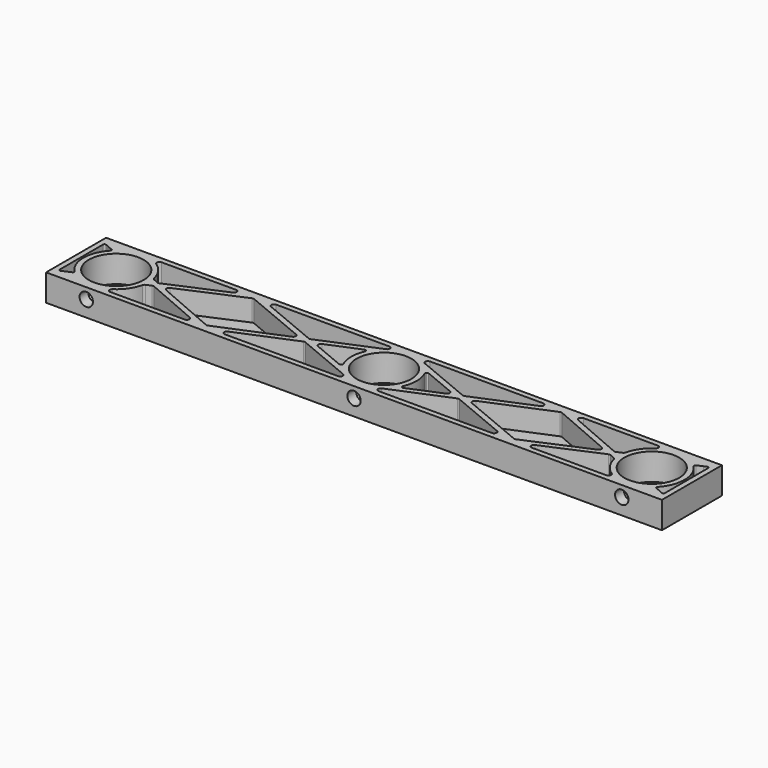
from build123d import *

# Parameters (mm, degrees)
F0_W          = 230
F0_H          = 28
F0_R          = 10.25
F1_DEPTH      = 2
F2_W          = 230
F2_H          = 28
F2_R          = 10.25
F3_DEPTH      = 8
F4_R          = 2.5
F5_DEPTH      = 10
F6_T3_DEPTH   = 8
F6_T6_DEPTH   = 15.8780595504
F6_S7_R       = 2.5
F6_T8_DEPTH   = 10
F6_T12_DEPTH  = 8
F6_T15_DEPTH  = 8
F6_T18_DEPTH  = 8
F6_T21_DEPTH  = 8
F6_T24_DEPTH  = 8
F6_T27_DEPTH  = 8
F6_T30_DEPTH  = 8
F6_T33_DEPTH  = 8
F6_T36_DEPTH  = 8
F6_T39_DEPTH  = 15.8780595504
F6_S41_R      = 2.5
F6_T42_DEPTH  = 10
F6_T45_DEPTH  = 9.0622287804
F6_T48_DEPTH  = 9.0622287804
F6_T51_DEPTH  = 8
F6_T54_DEPTH  = 8
F6_T57_DEPTH  = 9.0434782609
F6_T60_DEPTH  = 9.0434782609
F6_T63_DEPTH  = 8
F6_T66_DEPTH  = 8
F6_T69_DEPTH  = 8
F6_T72_DEPTH  = 8
F6_T75_DEPTH  = 8
F6_T78_DEPTH  = 8
F6_T81_DEPTH  = 8
F6_T84_DEPTH  = 8
F6_T87_DEPTH  = 9.2955278215
F6_T90_DEPTH  = 9.0810810811
F6_T93_DEPTH  = 9.0810810811
F6_T96_DEPTH  = 9.2955278215
F6_T99_DEPTH  = 9.0810810811
F6_T102_DEPTH = 9.2955278215
F6_T105_DEPTH = 9.0810810811
F6_T108_DEPTH = 9.2955278215
F6_T111_DEPTH = 9.0622287804
F6_T114_DEPTH = 9.0622287804
F6_T117_DEPTH = 9.0434782609
F6_T120_DEPTH = 9.0434782609
F6_T123_DEPTH = 15.8780595504
F6_S125_R     = 2.5
F6_T126_DEPTH = 10
F6_T129_DEPTH = 15.8780595504
F6_S130_R     = 2.5
F6_T131_DEPTH = 10
F7_R          = 0.5


# Not quite as in the source:
# - a fillet or chamfer that OpenCascade refuses, or shapes differently, is made with other operations: its cross-section is extruded or revolved along the edge and cut away or added


with BuildPart() as f1:
    # F0 (on Top) → F1 (new body)
    with BuildSketch(Plane.XY):
        Rectangle(F0_W, F0_H)
        with Locations((-100, 0)):
            Circle(F0_R, mode=Mode.SUBTRACT)
        Circle(F0_R, mode=Mode.SUBTRACT)
        with Locations((100, 0)):
            Circle(F0_R, mode=Mode.SUBTRACT)
    extrude(amount=F1_DEPTH)

    # F2 (on face) → F3 (join)
    with BuildSketch(Plane.XY.offset(2)):
        Rectangle(F2_W, F2_H)
        with BuildLine():
            Line((-87.9605861396, -2.261639648), (-85.25, -1.0894942903))
            Line((-85.25, -1.0894942903), (-60.0194555463, -12))
            Line((-60.0194555463, -12), (-97.5377855496, -12))
            ThreePointArc((-97.5377855496, -12), (-91.2659733511, -8.5894865095), (-87.9605861396, -2.261639648))
        make_face(mode=Mode.SUBTRACT)
        Polygon((-2.6102467372, -12), (-54.8897532628, -12), (-28.75, -1.0894942903), align=None, mode=Mode.SUBTRACT)
        Polygon((28.75, -1.0894942903), (54.8897532628, -12), (2.6102467372, -12), align=None, mode=Mode.SUBTRACT)
        with BuildLine():
            Line((85.25, -1.0894942903), (87.9605861396, -2.261639648))
            ThreePointArc((87.9605861396, -2.261639648), (91.2659733511, -8.5894865095), (97.5377855496, -12))
            Line((97.5377855496, -12), (60.0194555463, -12))
            Line((60.0194555463, -12), (85.25, -1.0894942903))
        make_face(mode=Mode.SUBTRACT)
        with BuildLine():
            Line((-113, -10.9105057097), (-113, 10.9105057097))
            Line((-113, 10.9105057097), (-111.274366755, 10.1642859281))
            Line((-111.274366755, 10.1642859281), (-108.3964347978, 8.9197748114))
            ThreePointArc((-108.3964347978, 8.9197748114), (-112.25, 0), (-108.3964347978, -8.9197748114))
            Line((-108.3964347978, -8.9197748114), (-111.274366755, -10.1642859281))
            Line((-111.274366755, -10.1642859281), (-113, -10.9105057097))
        make_face(mode=Mode.SUBTRACT)
        with Locations((-100, 0)):
            Circle(F2_R, mode=Mode.SUBTRACT)
        with BuildLine():
            Line((-85.25, 1.0894942903), (-87.9605861396, 2.261639648))
            ThreePointArc((-87.9605861396, 2.261639648), (-91.2659733511, 8.5894865095), (-97.5377855496, 12))
            Line((-97.5377855496, 12), (-60.0194555463, 12))
            Line((-60.0194555463, 12), (-85.25, 1.0894942903))
        make_face(mode=Mode.SUBTRACT)
        Polygon((-57.5, -10.9105057097), (-82.7305444537, 0), (-57.5, 10.9105057097), (-31.3602467372, 0), align=None, mode=Mode.SUBTRACT)
        with BuildLine():
            Line((-11.4782643731, 6.1195779714), (-11.0930792613, 5.196738641))
            ThreePointArc((-11.0930792613, 5.196738641), (-12.25, 0), (-11.0930792613, -5.196738641))
            Line((-11.0930792613, -5.196738641), (-11.4782643731, -6.1195779714))
            Line((-11.4782643731, -6.1195779714), (-26.1397532628, 0))
            Line((-26.1397532628, 0), (-11.4782643731, 6.1195779714))
        make_face(mode=Mode.SUBTRACT)
        Polygon((-28.75, 1.0894942903), (-54.8897532628, 12), (-2.6102467372, 12), align=None, mode=Mode.SUBTRACT)
        Circle(F2_R, mode=Mode.SUBTRACT)
        with BuildLine():
            Line((26.1397532628, 0), (11.4782643731, -6.1195779714))
            Line((11.4782643731, -6.1195779714), (11.0930792613, -5.196738641))
            ThreePointArc((11.0930792613, -5.196738641), (12.25, 0), (11.0930792613, 5.196738641))
            Line((11.0930792613, 5.196738641), (11.4782643731, 6.1195779714))
            Line((11.4782643731, 6.1195779714), (26.1397532628, 0))
        make_face(mode=Mode.SUBTRACT)
        Polygon((57.5, 10.9105057097), (82.7305444537, 0), (57.5, -10.9105057097), (31.3602467372, 0), align=None, mode=Mode.SUBTRACT)
        Polygon((28.75, 1.0894942903), (2.6102467372, 12), (54.8897532628, 12), align=None, mode=Mode.SUBTRACT)
        with Locations((100, 0)):
            Circle(F2_R, mode=Mode.SUBTRACT)
        with BuildLine():
            Line((111.274366755, 10.1642859281), (113, 10.9105057097))
            Line((113, 10.9105057097), (113, -10.9105057097))
            Line((113, -10.9105057097), (111.274366755, -10.1642859281))
            Line((111.274366755, -10.1642859281), (108.3964347978, -8.9197748114))
            ThreePointArc((108.3964347978, -8.9197748114), (112.25, 0), (108.3964347978, 8.9197748114))
            Line((108.3964347978, 8.9197748114), (111.274366755, 10.1642859281))
        make_face(mode=Mode.SUBTRACT)
        with BuildLine():
            ThreePointArc((97.5377855496, 12), (91.2659733511, 8.5894865095), (87.9605861396, 2.261639648))
            Line((87.9605861396, 2.261639648), (85.25, 1.0894942903))
            Line((85.25, 1.0894942903), (60.0194555463, 12))
            Line((60.0194555463, 12), (97.5377855496, 12))
        make_face(mode=Mode.SUBTRACT)
    extrude(amount=F3_DEPTH)

    # F4 (on face) → F5 (cut)
    with BuildSketch(Plane.XZ.offset(14)):
        with Locations((-100, 6)):
            Circle(F4_R)
        with Locations((0, 6)):
            Circle(F4_R)
        with Locations((100, 6)):
            Circle(F4_R)
    extrude(amount=-F5_DEPTH, mode=Mode.SUBTRACT)

    # F6: fillet of radius 1 on 40 edges, made by hand


with BuildPart() as f6_tool1:
    # F6_s2 → F6_t3 (new body)
    with BuildSketch(Plane.XY.offset(2)):
        with BuildLine():
            ThreePointArc((-93.1708391657, 10.1698113208), (-93.569962283, 11.2913857587), (-92.6133566486, 12))
            Line((-92.6133566486, 12), (-97.5377855496, 12))
            ThreePointArc((-97.5377855496, 12), (-95.2650436833, 11.2979063848), (-93.1708391657, 10.1698113208))
        make_face()
    extrude(amount=F6_T3_DEPTH)


with BuildPart() as f6_tool4:
    # F6_s5 → F6_t6 (new body)
    with BuildSketch(Plane.XY.offset(-5.8780595504)):
        with BuildLine():
            ThreePointArc((-93.1708391657, -10.1698113208), (-93.569962283, -11.2913857587), (-92.6133566486, -12))
            Line((-92.6133566486, -12), (-97.5377855496, -12))
            ThreePointArc((-97.5377855496, -12), (-95.2650436833, -11.2979063848), (-93.1708391657, -10.1698113208))
        make_face()
    extrude(amount=F6_T6_DEPTH)

    # F6_s7 → F6_t8 (cut, symmetric)
    with BuildSketch(Plane.XZ.offset(11.1)):
        with Locations((-100, 6)):
            Circle(F6_S7_R)
    extrude(amount=F6_T8_DEPTH, both=True, mode=Mode.SUBTRACT)

    split(bisect_by=Plane.XY.offset(2), keep=Keep.TOP)


with BuildPart() as f6_tool10:
    # F6_s11 → F6_t12 (new body)
    with BuildSketch(Plane.XY.offset(2)):
        with BuildLine():
            ThreePointArc((-64.454499942, 10.082142964), (-63.8721621366, 11.2026610027), (-64.8514110927, 12))
            Line((-64.8514110927, 12), (-60.0194555463, 12))
            Line((-60.0194555463, 12), (-64.454499942, 10.082142964))
        make_face()
    extrude(amount=F6_T12_DEPTH)


with BuildPart() as f6_tool13:
    # F6_s14 → F6_t15 (new body)
    with BuildSketch(Plane.XY.offset(2)):
        with BuildLine():
            ThreePointArc((-50.2829507005, 10.0771606696), (-50.878285688, 11.1964187741), (-49.8977655887, 12))
            Line((-49.8977655887, 12), (-54.8897532628, 12))
            Line((-54.8897532628, 12), (-50.2829507005, 10.0771606696))
        make_face()
    extrude(amount=F6_T15_DEPTH)


with BuildPart() as f6_tool16:
    # F6_s17 → F6_t18 (new body)
    with BuildSketch(Plane.XY.offset(2)):
        with BuildLine():
            ThreePointArc((-49.8977655887, -12), (-50.878285688, -11.1964187741), (-50.2829507005, -10.0771606696))
            Line((-50.2829507005, -10.0771606696), (-54.8897532628, -12))
            Line((-54.8897532628, -12), (-49.8977655887, -12))
        make_face()
    extrude(amount=F6_T18_DEPTH)


with BuildPart() as f6_tool19:
    # F6_s20 → F6_t21 (new body)
    with BuildSketch(Plane.XY.offset(2)):
        with BuildLine():
            ThreePointArc((-64.454499942, -10.082142964), (-63.8721621366, -11.2026610027), (-64.8514110927, -12))
            Line((-64.8514110927, -12), (-60.0194555463, -12))
            Line((-60.0194555463, -12), (-64.454499942, -10.082142964))
        make_face()
    extrude(amount=F6_T21_DEPTH)


with BuildPart() as f6_tool22:
    # F6_s23 → F6_t24 (new body)
    with BuildSketch(Plane.XY.offset(2)):
        with BuildLine():
            ThreePointArc((50.2829507005, 10.0771606696), (50.878285688, 11.1964187741), (49.8977655887, 12))
            Line((49.8977655887, 12), (54.8897532628, 12))
            Line((54.8897532628, 12), (50.2829507005, 10.0771606696))
        make_face()
    extrude(amount=F6_T24_DEPTH)


with BuildPart() as f6_tool25:
    # F6_s26 → F6_t27 (new body)
    with BuildSketch(Plane.XY.offset(2)):
        with BuildLine():
            ThreePointArc((50.2829507005, -10.0771606696), (50.878285688, -11.1964187741), (49.8977655887, -12))
            Line((49.8977655887, -12), (54.8897532628, -12))
            Line((54.8897532628, -12), (50.2829507005, -10.0771606696))
        make_face()
    extrude(amount=F6_T27_DEPTH)


with BuildPart() as f6_tool28:
    # F6_s29 → F6_t30 (new body)
    with BuildSketch(Plane.XY.offset(2)):
        with BuildLine():
            ThreePointArc((64.8514110927, 12), (63.8721621366, 11.2026610027), (64.454499942, 10.082142964))
            Line((64.454499942, 10.082142964), (60.0194555463, 12))
            Line((60.0194555463, 12), (64.8514110927, 12))
        make_face()
    extrude(amount=F6_T30_DEPTH)


with BuildPart() as f6_tool31:
    # F6_s32 → F6_t33 (new body)
    with BuildSketch(Plane.XY.offset(2)):
        with BuildLine():
            ThreePointArc((64.454499942, -10.082142964), (63.8721621366, -11.2026610027), (64.8514110927, -12))
            Line((64.8514110927, -12), (60.0194555463, -12))
            Line((60.0194555463, -12), (64.454499942, -10.082142964))
        make_face()
    extrude(amount=F6_T33_DEPTH)


with BuildPart() as f6_tool34:
    # F6_s35 → F6_t36 (new body)
    with BuildSketch(Plane.XY.offset(2)):
        with BuildLine():
            ThreePointArc((92.6133566486, 12), (93.569962283, 11.2913857587), (93.1708391657, 10.1698113208))
            ThreePointArc((93.1708391657, 10.1698113208), (95.2650436833, 11.2979063848), (97.5377855496, 12))
            Line((97.5377855496, 12), (92.6133566486, 12))
        make_face()
    extrude(amount=F6_T36_DEPTH)


with BuildPart() as f6_tool37:
    # F6_s38 → F6_t39 (new body)
    with BuildSketch(Plane.XY.offset(2)):
        with BuildLine():
            ThreePointArc((93.1708391657, -10.1698113208), (93.569962283, -11.2913857587), (92.6133566486, -12))
            Line((92.6133566486, -12), (97.5377855496, -12))
            ThreePointArc((97.5377855496, -12), (95.2650436833, -11.2979063848), (93.1708391657, -10.1698113208))
        make_face()
    extrude(amount=F6_T39_DEPTH)

    split(bisect_by=Plane.XY.offset(10), keep=Keep.BOTTOM)

    # F6_s41 → F6_t42 (cut, symmetric)
    with BuildSketch(Plane.XZ.offset(11.1)):
        with Locations((100, 6)):
            Circle(F6_S41_R)
    extrude(amount=F6_T42_DEPTH, both=True, mode=Mode.SUBTRACT)


with BuildPart() as f6_tool43:
    # F6_s44 → F6_t45 (new body)
    with BuildSketch(Plane.XY.offset(0.9377712196)):
        with BuildLine():
            ThreePointArc((-57.8899896639, 10.7418615307), (-57.4994488203, 10.8239842041), (-57.1078934015, 10.7468438251))
            Line((-57.1078934015, 10.7468438251), (-57.5, 10.9105057097))
            Line((-57.5, 10.9105057097), (-57.8899896639, 10.7418615307))
        make_face()
    extrude(amount=F6_T45_DEPTH)


with BuildPart() as f6_tool46:
    # F6_s47 → F6_t48 (new body)
    with BuildSketch(Plane.XY.offset(0.9377712196)):
        with BuildLine():
            ThreePointArc((-57.8899896639, -10.7418615307), (-57.4994488203, -10.8239842041), (-57.1078934015, -10.7468438251))
            Line((-57.1078934015, -10.7468438251), (-57.5, -10.9105057097))
            Line((-57.5, -10.9105057097), (-57.8899896639, -10.7418615307))
        make_face()
    extrude(amount=F6_T48_DEPTH)


with BuildPart() as f6_tool49:
    # F6_s50 → F6_t51 (new body)
    with BuildSketch(Plane.XY.offset(2)):
        with BuildLine():
            ThreePointArc((-33.5712159662, 0.9228393304), (-32.956401078, 0), (-33.5712159662, -0.9228393304))
            Line((-33.5712159662, -0.9228393304), (-31.3602467372, 0))
            Line((-31.3602467372, 0), (-33.5712159662, 0.9228393304))
        make_face()
    extrude(amount=F6_T51_DEPTH)


with BuildPart() as f6_tool52:
    # F6_s53 → F6_t54 (new body)
    with BuildSketch(Plane.XY.offset(2)):
        with BuildLine():
            ThreePointArc((-23.9287840338, -0.9228393304), (-24.543598922, 0), (-23.9287840338, 0.9228393304))
            Line((-23.9287840338, 0.9228393304), (-26.1397532628, 0))
            Line((-26.1397532628, 0), (-23.9287840338, -0.9228393304))
        make_face()
    extrude(amount=F6_T54_DEPTH)


with BuildPart() as f6_tool55:
    # F6_s56 → F6_t57 (new body)
    with BuildSketch(Plane.XY.offset(0.9565217391)):
        with BuildLine():
            ThreePointArc((-28.3648148882, 1.2502672065), (-28.75, 1.1731065369), (-29.1351851118, 1.2502672065))
            Line((-29.1351851118, 1.2502672065), (-28.75, 1.0894942903))
            Line((-28.75, 1.0894942903), (-28.3648148882, 1.2502672065))
        make_face()
    extrude(amount=F6_T57_DEPTH)


with BuildPart() as f6_tool58:
    # F6_s59 → F6_t60 (new body)
    with BuildSketch(Plane.XY.offset(0.9565217391)):
        with BuildLine():
            ThreePointArc((-29.1351851118, -1.2502672065), (-28.75, -1.1731065369), (-28.3648148882, -1.2502672065))
            Line((-28.3648148882, -1.2502672065), (-28.75, -1.0894942903))
            Line((-28.75, -1.0894942903), (-29.1351851118, -1.2502672065))
        make_face()
    extrude(amount=F6_T60_DEPTH)


with BuildPart() as f6_tool61:
    # F6_s62 → F6_t63 (new body)
    with BuildSketch(Plane.XY.offset(2)):
        with BuildLine():
            ThreePointArc((-80.608000058, -0.917857036), (-81.2110889073, 0), (-80.608000058, 0.917857036))
            Line((-80.608000058, 0.917857036), (-82.7305444537, 0))
            Line((-82.7305444537, 0), (-80.608000058, -0.917857036))
        make_face()
    extrude(amount=F6_T63_DEPTH)


with BuildPart() as f6_tool64:
    # F6_s65 → F6_t66 (new body)
    with BuildSketch(Plane.XY.offset(2)):
        with BuildLine():
            ThreePointArc((33.5712159662, -0.9228393304), (32.956401078, 0), (33.5712159662, 0.9228393304))
            Line((33.5712159662, 0.9228393304), (31.3602467372, 0))
            Line((31.3602467372, 0), (33.5712159662, -0.9228393304))
        make_face()
    extrude(amount=F6_T66_DEPTH)


with BuildPart() as f6_tool67:
    # F6_s68 → F6_t69 (new body)
    with BuildSketch(Plane.XY.offset(2)):
        with BuildLine():
            ThreePointArc((23.9287840338, 0.9228393304), (24.543598922, 0), (23.9287840338, -0.9228393304))
            Line((23.9287840338, -0.9228393304), (26.1397532628, 0))
            Line((26.1397532628, 0), (23.9287840338, 0.9228393304))
        make_face()
    extrude(amount=F6_T69_DEPTH)


with BuildPart() as f6_tool70:
    # F6_s71 → F6_t72 (new body)
    with BuildSketch(Plane.XY.offset(2)):
        with BuildLine():
            ThreePointArc((80.608000058, 0.917857036), (81.2110889073, 0), (80.608000058, -0.917857036))
            Line((80.608000058, -0.917857036), (82.7305444537, 0))
            Line((82.7305444537, 0), (80.608000058, 0.917857036))
        make_face()
    extrude(amount=F6_T72_DEPTH)


with BuildPart() as f6_tool73:
    # F6_s74 → F6_t75 (new body)
    with BuildSketch(Plane.XY.offset(2)):
        with BuildLine():
            ThreePointArc((7.2170492995, 10.0771606696), (6.621714312, 11.1964187741), (7.6022344113, 12))
            Line((7.6022344113, 12), (2.6102467372, 12))
            Line((2.6102467372, 12), (7.2170492995, 10.0771606696))
        make_face()
    extrude(amount=F6_T75_DEPTH)


with BuildPart() as f6_tool76:
    # F6_s77 → F6_t78 (new body)
    with BuildSketch(Plane.XY.offset(2)):
        with BuildLine():
            ThreePointArc((-7.2170492995, 10.0771606696), (-6.621714312, 11.1964187741), (-7.6022344113, 12))
            Line((-7.6022344113, 12), (-2.6102467372, 12))
            Line((-2.6102467372, 12), (-7.2170492995, 10.0771606696))
        make_face()
    extrude(amount=F6_T78_DEPTH)


with BuildPart() as f6_tool79:
    # F6_s80 → F6_t81 (new body)
    with BuildSketch(Plane.XY.offset(2)):
        with BuildLine():
            ThreePointArc((-7.6022344113, -12), (-6.621714312, -11.1964187741), (-7.2170492995, -10.0771606696))
            Line((-7.2170492995, -10.0771606696), (-2.6102467372, -12))
            Line((-2.6102467372, -12), (-7.6022344113, -12))
        make_face()
    extrude(amount=F6_T81_DEPTH)


with BuildPart() as f6_tool82:
    # F6_s83 → F6_t84 (new body)
    with BuildSketch(Plane.XY.offset(2)):
        with BuildLine():
            ThreePointArc((7.2170492995, -10.0771606696), (6.621714312, -11.1964187741), (7.6022344113, -12))
            Line((7.6022344113, -12), (2.6102467372, -12))
            Line((2.6102467372, -12), (7.2170492995, -10.0771606696))
        make_face()
    extrude(amount=F6_T84_DEPTH)


with BuildPart() as f6_tool85:
    # F6_s86 → F6_t87 (new body)
    with BuildSketch(Plane.XY.offset(0.7044721785)):
        with BuildLine():
            ThreePointArc((-87.4849424091, 2.0559558726), (-87.8564005011, 2.3338061064), (-88.0625194653, 2.7493741985))
            ThreePointArc((-88.0625194653, 2.7493741985), (-88.0090727024, 2.5060252479), (-87.9605861396, 2.261639648))
            Line((-87.9605861396, 2.261639648), (-87.4849424091, 2.0559558726))
        make_face()
    extrude(amount=F6_T87_DEPTH)


with BuildPart() as f6_tool88:
    # F6_s89 → F6_t90 (new body)
    with BuildSketch(Plane.XY.offset(0.9189189189)):
        with BuildLine():
            ThreePointArc((-84.8530888493, 1.2611315447), (-85.25, 1.1789885806), (-85.6469111507, 1.2611315447))
            Line((-85.6469111507, 1.2611315447), (-85.25, 1.0894942903))
            Line((-85.25, 1.0894942903), (-84.8530888493, 1.2611315447))
        make_face()
    extrude(amount=F6_T90_DEPTH)


with BuildPart() as f6_tool91:
    # F6_s92 → F6_t93 (new body)
    with BuildSketch(Plane.XY.offset(0.9189189189)):
        with BuildLine():
            ThreePointArc((-85.6469111507, -1.2611315447), (-85.25, -1.1789885806), (-84.8530888493, -1.2611315447))
            Line((-84.8530888493, -1.2611315447), (-85.25, -1.0894942903))
            Line((-85.25, -1.0894942903), (-85.6469111507, -1.2611315447))
        make_face()
    extrude(amount=F6_T93_DEPTH)


with BuildPart() as f6_tool94:
    # F6_s95 → F6_t96 (new body)
    with BuildSketch(Plane.XY.offset(0.7044721785)):
        with BuildLine():
            ThreePointArc((-88.0625194653, -2.7493741985), (-87.8564005011, -2.3338061064), (-87.4849424091, -2.0559558726))
            Line((-87.4849424091, -2.0559558726), (-87.9605861396, -2.261639648))
            ThreePointArc((-87.9605861396, -2.261639648), (-88.0090727024, -2.5060252479), (-88.0625194653, -2.7493741985))
        make_face()
    extrude(amount=F6_T96_DEPTH)


with BuildPart() as f6_tool97:
    # F6_s98 → F6_t99 (new body)
    with BuildSketch(Plane.XY.offset(0.9189189189)):
        with BuildLine():
            ThreePointArc((84.8530888493, -1.2611315447), (85.25, -1.1789885806), (85.6469111507, -1.2611315447))
            Line((85.6469111507, -1.2611315447), (85.25, -1.0894942903))
            Line((85.25, -1.0894942903), (84.8530888493, -1.2611315447))
        make_face()
    extrude(amount=F6_T99_DEPTH)


with BuildPart() as f6_tool100:
    # F6_s101 → F6_t102 (new body)
    with BuildSketch(Plane.XY.offset(0.7044721785)):
        with BuildLine():
            ThreePointArc((87.4849424091, -2.0559558726), (87.8564005011, -2.3338061064), (88.0625194653, -2.7493741985))
            ThreePointArc((88.0625194653, -2.7493741985), (88.0090727024, -2.5060252479), (87.9605861396, -2.261639648))
            Line((87.9605861396, -2.261639648), (87.4849424091, -2.0559558726))
        make_face()
    extrude(amount=F6_T102_DEPTH)


with BuildPart() as f6_tool103:
    # F6_s104 → F6_t105 (new body)
    with BuildSketch(Plane.XY.offset(0.9189189189)):
        with BuildLine():
            ThreePointArc((85.6469111507, 1.2611315447), (85.25, 1.1789885806), (84.8530888493, 1.2611315447))
            Line((84.8530888493, 1.2611315447), (85.25, 1.0894942903))
            Line((85.25, 1.0894942903), (85.6469111507, 1.2611315447))
        make_face()
    extrude(amount=F6_T105_DEPTH)


with BuildPart() as f6_tool106:
    # F6_s107 → F6_t108 (new body)
    with BuildSketch(Plane.XY.offset(0.7044721785)):
        with BuildLine():
            ThreePointArc((88.0625194653, 2.7493741985), (87.8564005011, 2.3338061064), (87.4849424091, 2.0559558726))
            Line((87.4849424091, 2.0559558726), (87.9605861396, 2.261639648))
            ThreePointArc((87.9605861396, 2.261639648), (88.0090727024, 2.5060252479), (88.0625194653, 2.7493741985))
        make_face()
    extrude(amount=F6_T108_DEPTH)


with BuildPart() as f6_tool109:
    # F6_s110 → F6_t111 (new body)
    with BuildSketch(Plane.XY.offset(0.9377712196)):
        with BuildLine():
            ThreePointArc((57.8899896639, -10.7418615307), (57.4994488203, -10.8239842041), (57.1078934015, -10.7468438251))
            Line((57.1078934015, -10.7468438251), (57.5, -10.9105057097))
            Line((57.5, -10.9105057097), (57.8899896639, -10.7418615307))
        make_face()
    extrude(amount=F6_T111_DEPTH)


with BuildPart() as f6_tool112:
    # F6_s113 → F6_t114 (new body)
    with BuildSketch(Plane.XY.offset(0.9377712196)):
        with BuildLine():
            ThreePointArc((57.8899896639, 10.7418615307), (57.4994488203, 10.8239842041), (57.1078934015, 10.7468438251))
            Line((57.1078934015, 10.7468438251), (57.5, 10.9105057097))
            Line((57.5, 10.9105057097), (57.8899896639, 10.7418615307))
        make_face()
    extrude(amount=F6_T114_DEPTH)


with BuildPart() as f6_tool115:
    # F6_s116 → F6_t117 (new body)
    with BuildSketch(Plane.XY.offset(0.9565217391)):
        with BuildLine():
            ThreePointArc((28.3648148882, -1.2502672065), (28.75, -1.1731065369), (29.1351851118, -1.2502672065))
            Line((29.1351851118, -1.2502672065), (28.75, -1.0894942903))
            Line((28.75, -1.0894942903), (28.3648148882, -1.2502672065))
        make_face()
    extrude(amount=F6_T117_DEPTH)


with BuildPart() as f6_tool118:
    # F6_s119 → F6_t120 (new body)
    with BuildSketch(Plane.XY.offset(0.9565217391)):
        with BuildLine():
            ThreePointArc((29.1351851118, 1.2502672065), (28.75, 1.1731065369), (28.3648148882, 1.2502672065))
            Line((28.3648148882, 1.2502672065), (28.75, 1.0894942903))
            Line((28.75, 1.0894942903), (29.1351851118, 1.2502672065))
        make_face()
    extrude(amount=F6_T120_DEPTH)


with BuildPart() as f6_tool121:
    # F6_s122 → F6_t123 (new body)
    with BuildSketch(Plane.XY.offset(2)):
        with BuildLine():
            ThreePointArc((-93.1708391657, -10.1698113208), (-93.569962283, -11.2913857587), (-92.6133566486, -12))
            Line((-92.6133566486, -12), (-97.5377855496, -12))
            ThreePointArc((-97.5377855496, -12), (-95.2650436833, -11.2979063848), (-93.1708391657, -10.1698113208))
        make_face()
    extrude(amount=F6_T123_DEPTH)

    split(bisect_by=Plane.XY.offset(10), keep=Keep.BOTTOM)

    # F6_s125 → F6_t126 (cut, symmetric)
    with BuildSketch(Plane.XZ.offset(11.1)):
        with Locations((-100, 6)):
            Circle(F6_S125_R)
    extrude(amount=F6_T126_DEPTH, both=True, mode=Mode.SUBTRACT)


with BuildPart() as f6_tool127:
    # F6_s128 → F6_t129 (new body)
    with BuildSketch(Plane.XY.offset(-5.8780595504)):
        with BuildLine():
            ThreePointArc((93.1708391657, -10.1698113208), (93.569962283, -11.2913857587), (92.6133566486, -12))
            Line((92.6133566486, -12), (97.5377855496, -12))
            ThreePointArc((97.5377855496, -12), (95.2650436833, -11.2979063848), (93.1708391657, -10.1698113208))
        make_face()
    extrude(amount=F6_T129_DEPTH)

    # F6_s130 → F6_t131 (cut, symmetric)
    with BuildSketch(Plane.XZ.offset(11.1)):
        with Locations((100, 6)):
            Circle(F6_S130_R)
    extrude(amount=F6_T131_DEPTH, both=True, mode=Mode.SUBTRACT)

    split(bisect_by=Plane.XY.offset(2), keep=Keep.TOP)


with BuildPart() as f1_1:
    add(f1.part)

    # F6_t133: union F6_tool1, F6_tool4, F6_tool10, F6_tool13, F6_tool16, F6_tool19, F6_tool22, F6_tool25, F6_tool28, F6_tool31, F6_tool34, F6_tool37, F6_tool43, F6_tool46, F6_tool49, F6_tool52, F6_tool55, F6_tool58, F6_tool61, F6_tool64, F6_tool67, F6_tool70, F6_tool73, F6_tool76, F6_tool79, F6_tool82, F6_tool85, F6_tool88, F6_tool91, F6_tool94, F6_tool97, F6_tool100, F6_tool103, F6_tool106, F6_tool109, F6_tool112, F6_tool115, F6_tool118, F6_tool121, F6_tool127
    add([f6_tool1.part, f6_tool4.part, f6_tool10.part, f6_tool13.part, f6_tool16.part, f6_tool19.part, f6_tool22.part, f6_tool25.part, f6_tool28.part, f6_tool31.part, f6_tool34.part, f6_tool37.part, f6_tool43.part, f6_tool46.part, f6_tool49.part, f6_tool52.part, f6_tool55.part, f6_tool58.part, f6_tool61.part, f6_tool64.part, f6_tool67.part, f6_tool70.part, f6_tool73.part, f6_tool76.part, f6_tool79.part, f6_tool82.part, f6_tool85.part, f6_tool88.part, f6_tool91.part, f6_tool94.part, f6_tool97.part, f6_tool100.part, f6_tool103.part, f6_tool106.part, f6_tool109.part, f6_tool112.part, f6_tool115.part, f6_tool118.part, f6_tool121.part, f6_tool127.part])

    # F7
    f7_edges = [f1_1.edges().sort_by_distance(p)[0] for p in [
        (-113, 10.910506, 6),
        (-108.396435, 8.919775, 6),
        (-108.396435, -8.919775, 6),
        (-113, -10.910506, 6),
        (113, 10.910506, 6),
        (108.396435, 8.919775, 6),
        (108.396435, -8.919775, 6),
        (113, -10.910506, 6),
        (-11.478264, 6.119578, 6),
        (-11.093079, 5.196739, 6),
        (-11.478264, -6.119578, 6),
        (-11.093079, -5.196739, 6),
        (11.093079, -5.196739, 6),
        (11.093079, 5.196739, 6),
        (11.478264, 6.119578, 6),
        (11.478264, -6.119578, 6),
    ]]
    fillet(f7_edges, radius=F7_R)


solid = f1_1.part
